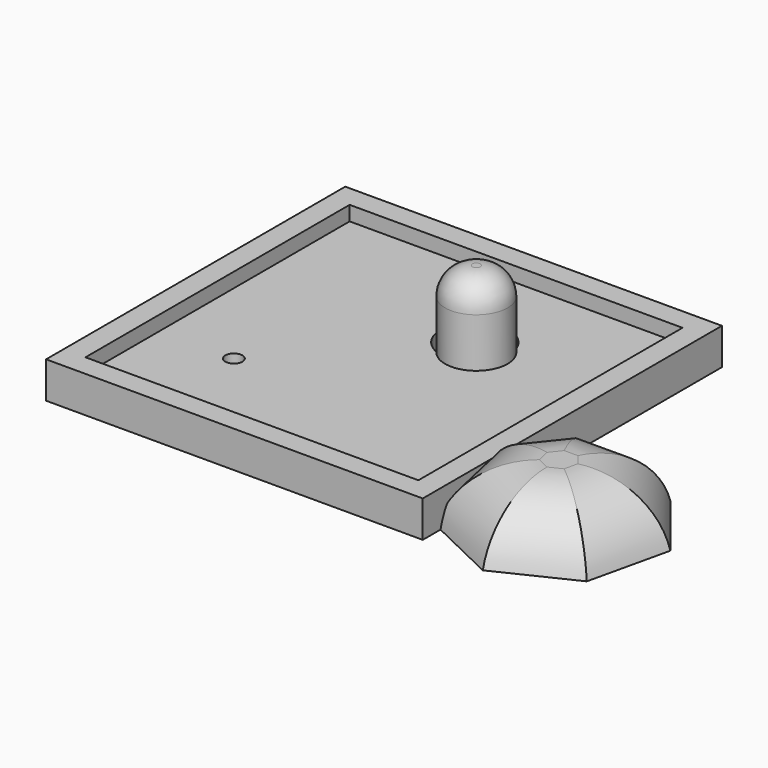
from build123d import *

# Parameters (mm, degrees)
F2_W          = 262.36371696
F2_H          = 260.4859247804
F3_DEPTH      = 25.4
F6_T          = -15.24
F8_D          = 47.533052
F9_R          = 21.7682047425
F10_DEPTH     = 68.58
F11_R         = 19.0095175901
F13_DEPTH     = 40.64
F14_T1_DEPTH  = 309.8053408432
F14_T3_DEPTH  = 309.8053408432
F14_T5_DEPTH  = 309.8053408432
F14_T7_DEPTH  = 309.8053408432
F14_T9_DEPTH  = 309.8053408432
F14_T11_DEPTH = 309.8053408432
F14_T13_DEPTH = 309.8053408432
F15_D         = 11.9634


# Not quite as in the source:
# - a fillet or chamfer that OpenCascade refuses, or shapes differently, is made with other operations: its cross-section is extruded or revolved along the edge and cut away or added
# - the program builds the solid bodies; features that only make, move or delete a surface that nothing else refers to are left out


with BuildPart() as f3:
    # F2 (on Top) → F3 (new body)
    with BuildSketch(Plane.XY):
        with Locations((15.5406966805, -5.9967003763)):
            Rectangle(F2_W, F2_H)
    extrude(amount=F3_DEPTH)

    # F6
    f6_openings = [f3.faces().sort_by_distance(p)[0] for p in [
        (15.540697, -5.9967, 25.4),
    ]]
    offset(amount=F6_T, openings=f6_openings)

    # F8 (through all)
    with Locations(Plane.XY.offset(15.24)):
        with Locations((41.753936559, 40.3167158365)):
            Hole(F8_D / 2)

    # F15 (through all)
    with Locations(Plane(origin=(0, 0, 0), x_dir=(1, 0, 0), z_dir=(0, 0, -1))):
        with Locations((-48.6491061747, 56.4698465168)):
            Hole(F15_D / 2)


with BuildPart() as f10:
    # F9 (on Top) → F10 (new body)
    with BuildSketch(Plane.XY):
        with Locations((49.7697815299, 31.5912254155)):
            Circle(F9_R)
    extrude(amount=F10_DEPTH)

    # F11
    f11_edges = [f10.edges().sort_by_distance(p)[0] for p in [
        (28.001577, 31.591225, 68.58),
    ]]
    fillet(f11_edges, radius=F11_R)


with BuildPart() as f13:
    # F12 (on Top) → F13 (new body)
    with BuildSketch(Plane.XY):
        Polygon((223.6656961674, -16.6721306741), (165.6090202099, -16.6721306741), (129.4112748206, -62.0626677051), (142.330100577, -118.6637415846), (194.6373581886, -143.8535892298), (246.9446158002, -118.6637415846), (259.8634415567, -62.0626677051), align=None)
    extrude(amount=F13_DEPTH)

    # F14: fillet of radius 51.5096605668 on 7 edges, made by hand

    # F14_s2 → F14_t1 (cut)
    with BuildSketch(Plane(origin=(209.7538690392, -263.0230324464, 0), x_dir=(0, 0, 1), z_dir=(-0.6234898019, 0.7818314825, 0))):
        with BuildLine():
            ThreePointArc((0, 164.4739793612), (29.2123656917, 146.4766234639), (40.64, 114.1242463841))
            Line((40.64, 114.1242463841), (40.64, 164.4739793612))
            Line((40.64, 164.4739793612), (0, 164.4739793612))
        make_face()
    extrude(amount=F14_T1_DEPTH, mode=Mode.SUBTRACT)

    # F14_s4 → F14_t3 (cut)
    with BuildSketch(Plane.YZ.offset(39.734687767)):
        with BuildLine():
            ThreePointArc((-16.6721306741, 0), (-34.6694865714, 29.2123656917), (-67.0218636513, 40.64))
            Line((-67.0218636513, 40.64), (-16.6721306741, 40.64))
            Line((-16.6721306741, 40.64), (-16.6721306741, 0))
        make_face()
    extrude(amount=F14_T3_DEPTH, mode=Mode.SUBTRACT)

    # F14_s6 → F14_t5 (cut)
    with BuildSketch(Plane(origin=(134.7330729996, 168.9499297129, 0), x_dir=(0, 0, 1), z_dir=(-0.6234898019, -0.7818314825, 0))):
        with BuildLine():
            ThreePointArc((0, -139.8732492313), (29.2123656917, -157.8706051286), (40.64, -190.2229822085))
            Line((40.64, -190.2229822085), (40.64, -139.8732492313))
            Line((40.64, -139.8732492313), (0, -139.8732492313))
        make_face()
    extrude(amount=F14_T5_DEPTH, mode=Mode.SUBTRACT)

    # F14_s8 → F14_t7 (cut)
    with BuildSketch(Plane(origin=(-8.1378103287, 35.654076641, 0), x_dir=(0, 0, 1), z_dir=(0.222520934, -0.9749279122, 0))):
        with BuildLine():
            ThreePointArc((0, -112.356421192), (29.2123656917, -130.3537770893), (40.64, -162.7061541692))
            Line((40.64, -162.7061541692), (40.64, -112.356421192))
            Line((40.64, -112.356421192), (0, -112.356421192))
        make_face()
    extrude(amount=F14_T7_DEPTH, mode=Mode.SUBTRACT)

    # F14_s10 → F14_t9 (cut)
    with BuildSketch(Plane(origin=(48.5144030923, -23.3633051759, 0), x_dir=(0, 0, 1), z_dir=(0.9009688679, -0.4338837391, 0))):
        with BuildLine():
            ThreePointArc((0, 45.1576206892), (29.2123656917, 27.1602647919), (40.64, -5.1921122879))
            Line((40.64, -5.1921122879), (40.64, 45.1576206892))
            Line((40.64, 45.1576206892), (0, 45.1576206892))
        make_face()
    extrude(amount=F14_T9_DEPTH, mode=Mode.SUBTRACT)

    # F14_s12 → F14_t11 (cut)
    with BuildSketch(Plane(origin=(-11.6476042219, -5.6091905632, 0), x_dir=(0, 0, 1), z_dir=(0.9009688679, 0.4338837391, 0))):
        with BuildLine():
            ThreePointArc((0, 214.0575901749), (29.2123656917, 196.0602342776), (40.64, 163.7078571978))
            Line((40.64, 163.7078571978), (40.64, 214.0575901749))
            Line((40.64, 214.0575901749), (0, 214.0575901749))
        make_face()
    extrude(amount=F14_T11_DEPTH, mode=Mode.SUBTRACT)

    # F14_s14 → F14_t13 (cut)
    with BuildSketch(Plane(origin=(-41.5252055305, -181.9338127472, 0), x_dir=(0, 0, 1), z_dir=(0.222520934, 0.9749279122, 0))):
        with BuildLine():
            ThreePointArc((0, 267.1583653108), (29.2123656917, 249.1610094135), (40.64, 216.8086323337))
            Line((40.64, 216.8086323337), (40.64, 267.1583653108))
            Line((40.64, 267.1583653108), (0, 267.1583653108))
        make_face()
    extrude(amount=F14_T13_DEPTH, mode=Mode.SUBTRACT)


solid = Compound([f3.part, f10.part, f13.part])
